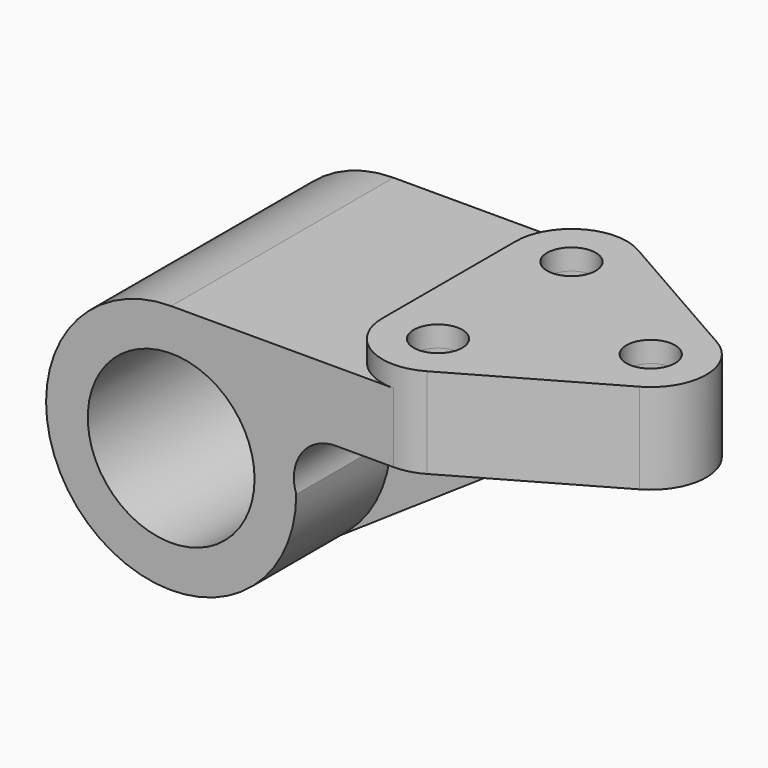
from build123d import *

# Parameters (mm, degrees)
F0_R     = 19.05
F1_DEPTH = 31.75
F3_R     = 5.5626
F4_DEPTH = 4.7752
F5_DEPTH = 57.151
F6_DEPTH = 15.875
F7_DEPTH = 4.7625
F8_DEPTH = 57.151


with BuildPart() as f1:
    # F0 (on Front) → F1 (new body, symmetric)
    with BuildSketch(Plane.XZ):
        with BuildLine():
            Line((37.5552561211, 28.575), (0, 28.575))
            ThreePointArc((0, 28.575), (-27.3235693319, -8.3638020041), (15.9950252975, -23.6788891364))
            ThreePointArc((15.9950252975, -23.6788891364), (25.2347822744, -13.4065800472), (28.575, 0))
            ThreePointArc((28.575, 0), (29.7781261877, 8.674261314), (37.5552561211, 12.7))
            Line((37.5552561211, 12.7), (69.85, 12.7))
            Line((69.85, 12.7), (96.3054561211, 12.7))
            Line((96.3054561211, 12.7), (96.3054561211, 28.575))
            Line((96.3054561211, 28.575), (37.5552561211, 28.575))
        make_face()
        Circle(F0_R, mode=Mode.SUBTRACT)
    extrude(amount=F1_DEPTH, both=True)

    # F3 (on offset) → F4 (join)
    with BuildSketch(Plane.XY.offset(28.575)):
        with BuildLine():
            Line((90.4493554441, 11.0277214642), (57.0991554441, 30.0777214642))
            ThreePointArc((57.0991554441, 30.0777214642), (44.4246284085, 30.0338352623), (38.1, 19.05))
            Line((38.1, 19.05), (38.1, -19.05))
            ThreePointArc((38.1, -19.05), (44.4246284085, -30.0338352623), (57.0991554441, -30.0777214642))
            Line((57.0991554441, -30.0777214642), (90.4493554441, -11.0277214642))
            ThreePointArc((90.4493554441, -11.0277214642), (96.8502, 0), (90.4493554441, 11.0277214642))
        make_face()
        with Locations((50.8, -19.05)):
            Circle(F3_R, mode=Mode.SUBTRACT)
        with Locations((50.8, 19.05)):
            Circle(F3_R, mode=Mode.SUBTRACT)
        with Locations((84.1502, 0)):
            Circle(F3_R, mode=Mode.SUBTRACT)
    extrude(amount=F4_DEPTH)

    # F5 (cut, through all): faces of the model
    f5_faces = [f1.faces().sort_by_distance(p)[0] for p in [
        (82.3575672844, 23.549714807, 28.575),
        (82.3575672844, -23.549714807, 28.575),
    ]]
    extrude(f5_faces, amount=-F5_DEPTH, mode=Mode.SUBTRACT)

    # F6 (add): a face of the model
    f6_faces = [f1.faces().sort_by_distance(p)[0] for p in [
        (96.5237592602, 0, 28.575),
    ]]
    extrude(f6_faces, amount=F6_DEPTH)

    # F0 (on Front) → F7 (join, symmetric)
    with BuildSketch(Plane.XZ):
        with BuildLine():
            ThreePointArc((28.575, 0), (25.2347822744, -13.4065800472), (15.9950252975, -23.6788891364))
            Line((15.9950252975, -23.6788891364), (69.85, 12.7))
            Line((69.85, 12.7), (37.5552561211, 12.7))
            ThreePointArc((37.5552561211, 12.7), (29.7781261877, 8.674261314), (28.575, 0))
        make_face()
    extrude(amount=F7_DEPTH, both=True)

    # F8 (cut, through all): faces of the model
    f8_faces = [f1.faces().sort_by_distance(p)[0] for p in [
        (50.8, -19.05, 28.575),
        (50.8, 19.05, 28.575),
        (84.1502, 0, 28.575),
    ]]
    extrude(f8_faces, amount=-F8_DEPTH, mode=Mode.SUBTRACT)


solid = f1.part
